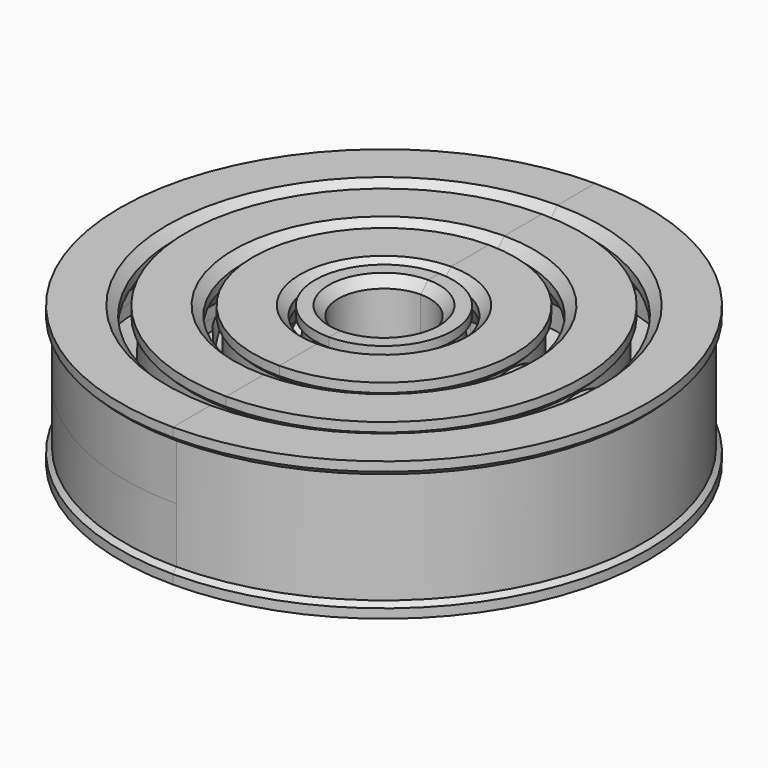
from build123d import *
from build123d import SkipClean  # not in build123d's __all__

# Parameters (mm, degrees)
F4_ANGLE_BACK = 90
F4_ANGLE      = 180
F5_ANGLE_BACK = 90
F5_ANGLE      = 180
F6_SIZE       = 0.8
F6_2_SIZE     = 0.8
F6_3_SIZE     = 0.8
F6_4_SIZE     = 0.8


with BuildPart() as f4:
    # F3 (on Front) → F4 (revolve)
    with BuildSketch(Plane.XZ, mode=Mode.PRIVATE) as f4_sk:
        Polygon((4, -4.7327868556), (4, -6.0380705357), (5.6, -6.0380705357), (5.6, -4.8380705357), (5.6, -4.7327868556), align=None)
        with BuildLine():
            Line((5.6, -4.7327868556), (5.6, 0))
            ThreePointArc((5.6, 0), (5.1845925587, -2.1166010489), (4, -3.9191835885))
            Line((4, -3.9191835885), (4, -4.7327868556))
            Line((4, -4.7327868556), (5.6, -4.7327868556))
        make_face()
        with BuildLine():
            Line((5.6, 0), (4, 0))
            Line((4, 0), (4, -3.9191835885))
            ThreePointArc((4, -3.9191835885), (5.1845925587, -2.1166010489), (5.6, 0))
        make_face()
        Polygon((5.6, -4.8380705357), (5.6, -6.0380705357), (6, -6.0380705357), (6, -5.2380705357), align=None)
    revolve(f4_sk.sketch.rotate(Axis((0, 0, -3.0190352678), (0, 0, -1)), -F4_ANGLE_BACK), axis=Axis((0, 0, -3.0190352678), (0, 0, -1)), revolution_arc=F4_ANGLE)

    # F3 (on Front) → F5 (revolve)
    with BuildSketch(Plane.XZ, mode=Mode.PRIVATE) as f5_sk:
        Polygon((8.9, 0), (5.6, 0), (5.6, -4.7327868556), (8.9, -0.8), align=None)
        with BuildLine():
            Line((5.6, -4.7327868556), (5.6, 0))
            ThreePointArc((5.6, 0), (5.1845925587, -2.1166010489), (4, -3.9191835885))
            Line((4, -3.9191835885), (4, -4.7327868556))
            Line((4, -4.7327868556), (5.6, -4.7327868556))
        make_face()
    revolve(f5_sk.sketch.rotate(Axis((10.2, 0, 0), (1, 0, 0)), -F5_ANGLE_BACK), axis=Axis((10.2, 0, 0), (1, 0, 0)), revolution_arc=F5_ANGLE)

    # F6#4
    f6_4_edges = [f4.edges().sort_by_distance(p)[0] for p in [
        (4, 0, -6.038071),
    ]]
    chamfer(f6_4_edges, length=F6_4_SIZE)



with BuildPart() as f4b:
    # F3 (on Front) → F4, piece 2 (revolve)
    with BuildSketch(Plane.XZ, mode=Mode.PRIVATE) as f4_sk:
        with BuildLine():
            Line((6.5, -4.4380705357), (6.5, -6.0380705357))
            Line((6.5, -6.0380705357), (9.1946562854, -6.0380705357))
            ThreePointArc((9.1946562854, -6.0380705357), (9.5844693325, -5.3979577262), (9.9297899565, -4.7327868556))
            ThreePointArc((9.9297899565, -4.7327868556), (10.7291120211, -2.4261399876), (11, 0))
            Line((11, 0), (9.4, 0))
            Line((9.4, 0), (9.4, -0.9819851171))
            Line((9.4, -0.9819851171), (6.5, -4.4380705357))
        make_face()
        with BuildLine():
            ThreePointArc((9.9297899565, -4.7327868556), (9.5844693325, -5.3979577262), (9.1946562854, -6.0380705357))
            Line((9.1946562854, -6.0380705357), (11, -6.0380705357))
            Line((11, -6.0380705357), (11, -4.8380705357))
            Line((11, -4.8380705357), (11, -4.7327868556))
            Line((11, -4.7327868556), (9.9297899565, -4.7327868556))
        make_face()
        with BuildLine():
            ThreePointArc((11, 0), (10.7291120211, -2.4261399876), (9.9297899565, -4.7327868556))
            Line((9.9297899565, -4.7327868556), (11, -4.7327868556))
            Line((11, -4.7327868556), (11, 0))
        make_face()
        Polygon((11, -4.8380705357), (11, -6.0380705357), (11.4, -6.0380705357), (11.4, -5.2380705357), align=None)
    revolve(f4_sk.sketch.rotate(Axis((0, 0, -3.0190352678), (0, 0, -1)), -F4_ANGLE_BACK), axis=Axis((0, 0, -3.0190352678), (0, 0, -1)), revolution_arc=F4_ANGLE)

    # F3 (on Front) → F5, piece 2 (revolve)
    with BuildSketch(Plane.XZ, mode=Mode.PRIVATE) as f5_sk:
        Polygon((14.3, 0), (11, 0), (11, -4.7327868556), (14.3, -0.8), align=None)
        with BuildLine():
            ThreePointArc((11, 0), (10.7291120211, -2.4261399876), (9.9297899565, -4.7327868556))
            Line((9.9297899565, -4.7327868556), (11, -4.7327868556))
            Line((11, -4.7327868556), (11, 0))
        make_face()
    revolve(f5_sk.sketch.rotate(Axis((10.2, 0, 0), (1, 0, 0)), -F5_ANGLE_BACK), axis=Axis((10.2, 0, 0), (1, 0, 0)), revolution_arc=F5_ANGLE)

    # F6
    f6_edges = [f4b.edges().sort_by_distance(p)[0] for p in [
        (6.5, 0, -6.038071),
    ]]
    chamfer(f6_edges, length=F6_SIZE)


with BuildPart() as f4c:
    # F3 (on Front) → F4, piece 3 (revolve)
    with BuildSketch(Plane.XZ, mode=Mode.PRIVATE) as f4_sk:
        with BuildLine():
            ThreePointArc((16.1195759429, -4.7327868556), (16.6290239618, -2.3907241747), (16.8, 0))
            Line((16.8, 0), (15.2, 0))
            Line((15.2, 0), (15.2, -0.9819851171))
            Line((15.2, -0.9819851171), (12.3, -4.4380705357))
            Line((12.3, -4.4380705357), (12.3, -6.0380705357))
            Line((12.3, -6.0380705357), (15.6774265811, -6.0380705357))
            ThreePointArc((15.6774265811, -6.0380705357), (15.9118912688, -5.3899644016), (16.1195759429, -4.7327868556))
        make_face()
        with BuildLine():
            Line((16.8, -4.7327868556), (16.8, 0))
            ThreePointArc((16.8, 0), (16.6290239618, -2.3907241747), (16.1195759429, -4.7327868556))
            Line((16.1195759429, -4.7327868556), (16.8, -4.7327868556))
        make_face()
        with BuildLine():
            Line((16.8, -4.8380705357), (16.8, -4.7327868556))
            Line((16.8, -4.7327868556), (16.1195759429, -4.7327868556))
            ThreePointArc((16.1195759429, -4.7327868556), (15.9118912688, -5.3899644016), (15.6774265811, -6.0380705357))
            Line((15.6774265811, -6.0380705357), (16.8, -6.0380705357))
            Line((16.8, -6.0380705357), (16.8, -4.8380705357))
        make_face()
        Polygon((17.2, -5.2380705357), (16.8, -4.8380705357), (16.8, -6.0380705357), (17.2, -6.0380705357), align=None)
    revolve(f4_sk.sketch.rotate(Axis((0, 0, -3.0190352678), (0, 0, -1)), -F4_ANGLE_BACK), axis=Axis((0, 0, -3.0190352678), (0, 0, -1)), revolution_arc=F4_ANGLE)

    # F3 (on Front) → F5, piece 3 (revolve)
    with BuildSketch(Plane.XZ, mode=Mode.PRIVATE) as f5_sk:
        Polygon((20.1, -0.8), (20.1, 0), (16.8, 0), (16.8, -4.7327868556), align=None)
        with BuildLine():
            Line((16.8, -4.7327868556), (16.8, 0))
            ThreePointArc((16.8, 0), (16.6290239618, -2.3907241747), (16.1195759429, -4.7327868556))
            Line((16.1195759429, -4.7327868556), (16.8, -4.7327868556))
        make_face()
    revolve(f5_sk.sketch.rotate(Axis((10.2, 0, 0), (1, 0, 0)), -F5_ANGLE_BACK), axis=Axis((10.2, 0, 0), (1, 0, 0)), revolution_arc=F5_ANGLE)

    # F6#2
    f6_2_edges = [f4c.edges().sort_by_distance(p)[0] for p in [
        (12.3, 0, -6.038071),
    ]]
    chamfer(f6_2_edges, length=F6_2_SIZE)


with BuildPart() as f4d:
    # F3 (on Front) → F4, piece 4 (revolve)
    with BuildSketch(Plane.XZ, mode=Mode.PRIVATE) as f4_sk:
        with BuildLine():
            ThreePointArc((22.0988852339, -4.7327868556), (22.4743721412, -2.3796211583), (22.6, 0))
            Line((22.6, 0), (21, 0))
            Line((21, 0), (21, -0.9819851171))
            Line((21, -0.9819851171), (18.1, -4.4380705357))
            Line((18.1, -4.4380705357), (18.1, -6.0380705357))
            Line((18.1, -6.0380705357), (21.7784688214, -6.0380705357))
            ThreePointArc((21.7784688214, -6.0380705357), (21.9483824255, -5.3878111423), (22.0988852339, -4.7327868556))
        make_face()
        with BuildLine():
            Line((22.6, -4.7327868556), (22.6, 0))
            ThreePointArc((22.6, 0), (22.4743721412, -2.3796211583), (22.0988852339, -4.7327868556))
            Line((22.0988852339, -4.7327868556), (22.6, -4.7327868556))
        make_face()
        with BuildLine():
            Line((22.6, -4.8380705357), (22.6, -4.7327868556))
            Line((22.6, -4.7327868556), (22.0988852339, -4.7327868556))
            ThreePointArc((22.0988852339, -4.7327868556), (21.9483824255, -5.3878111423), (21.7784688214, -6.0380705357))
            Line((21.7784688214, -6.0380705357), (22.6, -6.0380705357))
            Line((22.6, -6.0380705357), (22.6, -4.8380705357))
        make_face()
        Polygon((23, -5.2380705357), (22.6, -4.8380705357), (22.6, -6.0380705357), (23, -6.0380705357), align=None)
    revolve(f4_sk.sketch.rotate(Axis((0, 0, -3.0190352678), (0, 0, -1)), -F4_ANGLE_BACK), axis=Axis((0, 0, -3.0190352678), (0, 0, -1)), revolution_arc=F4_ANGLE)

    # F6#3
    f6_3_edges = [f4d.edges().sort_by_distance(p)[0] for p in [
        (18.1, 0, -6.038071),
    ]]
    chamfer(f6_3_edges, length=F6_3_SIZE)


with BuildPart() as f4_1:
    add(f4.part, clean=False)

    with SkipClean():  # cleaning this boolean's faces spoils the solid; the shape is the same uncleaned
        add(f4b.part)  # F7 merges F4b

    with SkipClean():  # cleaning this boolean's faces spoils the solid; the shape is the same uncleaned
        add(f4c.part)  # F7 merges F4c

    with SkipClean():  # cleaning this boolean's faces spoils the solid; the shape is the same uncleaned
        add(f4d.part)  # F7 merges F4d
    # F7: F4, F4b, F4c, F4d across face
    with SkipClean():  # cleaning this boolean's faces spoils the solid; the shape is the same uncleaned
        add(f4.part.mirror(Plane(origin=(4.7488950851, 0, 0), x_dir=(1, 0, 0), z_dir=(0, 0, 1))), clean=False)
        add(f4b.part.mirror(Plane(origin=(4.7488950851, 0, 0), x_dir=(1, 0, 0), z_dir=(0, 0, 1))), clean=False)
        add(f4c.part.mirror(Plane(origin=(4.7488950851, 0, 0), x_dir=(1, 0, 0), z_dir=(0, 0, 1))), clean=False)
        add(f4d.part.mirror(Plane(origin=(4.7488950851, 0, 0), x_dir=(1, 0, 0), z_dir=(0, 0, 1))), clean=False)

    # F8: F4 across face


with BuildPart() as f4_2:
    add(f4_1.part, clean=False)
    with SkipClean():  # cleaning this boolean's faces spoils the solid; the shape is the same uncleaned
        add(f4_1.part.mirror(Plane(origin=(0, 4.8580369973, 0), x_dir=(0, -1, 0), z_dir=(-1, 0, 0))), clean=False)


solid = f4_2.part
